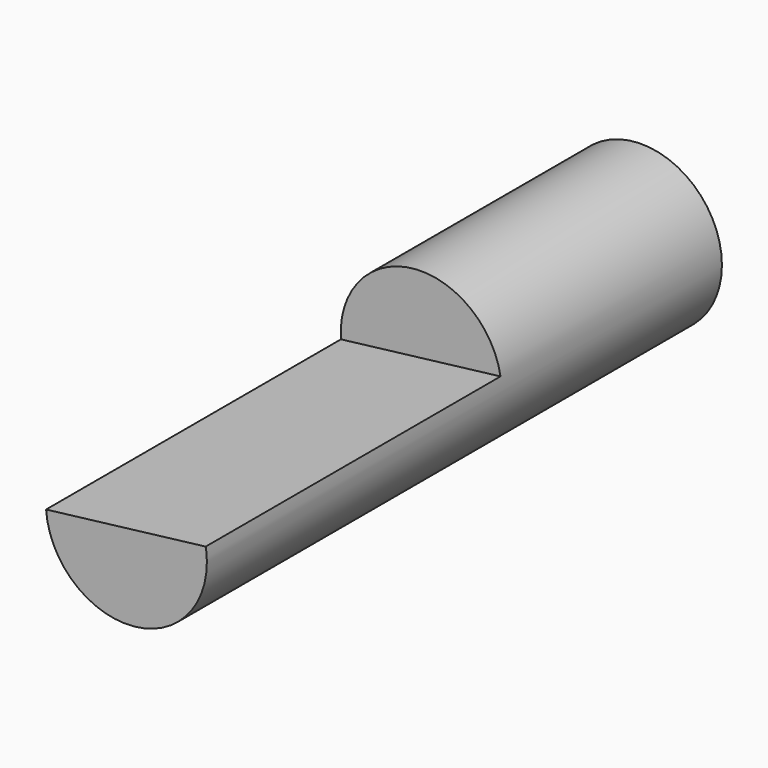
from build123d import *

# Parameters (mm, degrees)
F0_R     = 3.175
F1_DEPTH = 25.4
F4_W     = 8.473996073
F4_H     = 15.0644984096
F5_DEPTH = 25.4


with BuildPart() as f1:
    # F0 (on Front) → F1 (new body)
    with BuildSketch(Plane.XZ):
        with Locations((-45.5696061254, 7.3693422601)):
            Circle(F0_R)
    extrude(amount=F1_DEPTH)

    # F4 (on line) → F5 (cut)
    with BuildSketch(Plane(origin=(-1.5477918404, 0, 12.8342080993), x_dir=(0.9928063231, 0, 0.1197313862), z_dir=(0.1197313862, 0, -0.9928063231))):
        with Locations((-45.0706910342, 18.3933349326)):
            Rectangle(F4_W, F4_H)
    extrude(amount=-F5_DEPTH, mode=Mode.SUBTRACT)


solid = f1.part
